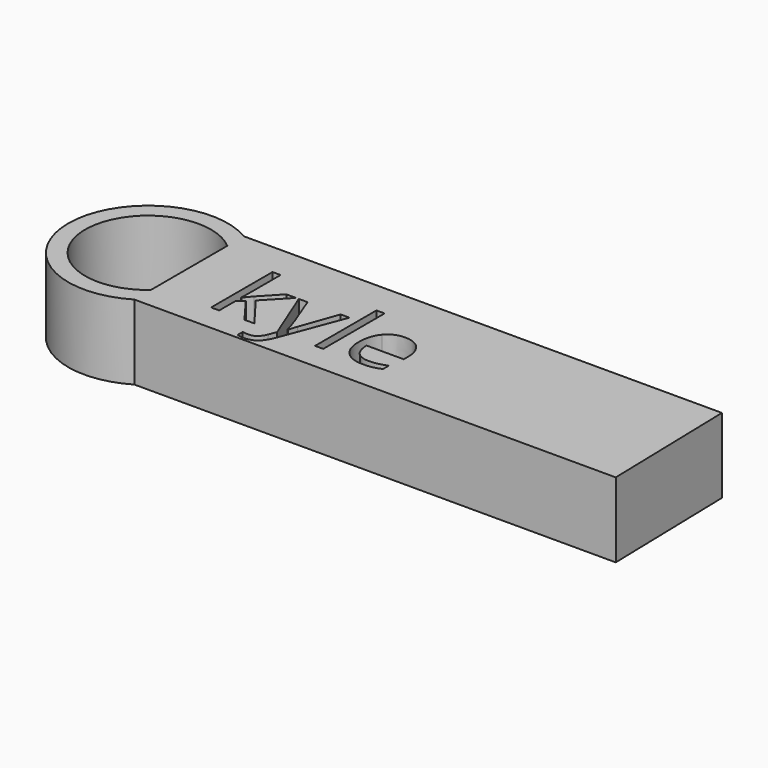
from build123d import *

# Parameters (mm, degrees)
F0_W     = 1.390167144
F0_H     = 13.0257857824
F1_DEPTH = 12.7


with BuildPart() as f1:
    # F0 (on Top) → F1 (new body)
    with BuildSketch(Plane.XY):
        with BuildLine():
            Line((-43.1278555505, 8.1087965258), (-43.1278555505, 11.6189617885))
            ThreePointArc((-43.1278555505, 11.6189617885), (-63.6173153539, 0), (-43.1278555505, -11.6189617885))
            Line((-43.1278555505, -11.6189617885), (-43.1278555505, -8.1087965258))
            ThreePointArc((-43.1278555505, -8.1087965258), (-60.7580848758, 0), (-43.1278555505, 8.1087965258))
        make_face()
        Polygon((37.9903619809, 11.6189617885), (-43.1278555505, 11.6189617885), (-43.1278555505, 8.1087965258), (-43.1278555505, -8.1087965258), (-43.1278555505, -11.6189617885), (38.5659746826, -11.6189617885), align=None)
        with BuildLine():
            Line((-22.5185390528, -7.0921576955), (-26.2202943379, 2.1327664737))
            Line((-26.2202943379, 2.1327664737), (-24.7283423163, 2.1327664737))
            Line((-24.7283423163, 2.1327664737), (-22.7194302586, -3.0984405247))
            add(Edge.make_bspline(
                [(-22.7194302586, -3.0984405247), (-22.0605071037, -4.8903900802), (-21.899794139, -5.6859192551)],
                knots=[0, 0, 0, 1, 1, 1], degree=2))
            Line((-21.899794139, -5.6859192551), (-21.8328304038, -5.6859192551))
            add(Edge.make_bspline(
                [(-21.8328304038, -5.6859192551), (-21.7256884274, -5.2573513494), (-21.377477004, -4.223431277)],
                knots=[0, 0, 0, 1, 1, 1], degree=2))
            add(Edge.make_bspline(
                [(-21.377477004, -4.223431277), (-21.0292655807, -3.1895112047), (-19.1033885547, 2.1327664737)],
                knots=[0, 0, 0, 1, 1, 1], degree=2))
            Line((-19.1033885547, 2.1327664737), (-17.6141150825, 2.1327664737))
            Line((-17.6141150825, 2.1327664737), (-21.5569398145, -8.3135762266))
            add(Edge.make_bspline(
                [(-21.5569398145, -8.3135762266), (-22.1435421354, -9.8617777858), (-22.9256785632, -10.5113260178)],
                knots=[0, 0, 0, 1, 1, 1], degree=2))
            add(Edge.make_bspline(
                [(-22.9256785632, -10.5113260178), (-23.707814991, -11.1608742498), (-24.8461984904, -11.1608742498)],
                knots=[0, 0, 0, 1, 1, 1], degree=2))
            add(Edge.make_bspline(
                [(-24.8461984904, -11.1608742498), (-25.4836932501, -11.1608742498), (-26.1024381638, -11.0162325816)],
                knots=[0, 0, 0, 1, 1, 1], degree=2))
            Line((-26.1024381638, -11.0162325816), (-26.1024381638, -9.9046345763))
            add(Edge.make_bspline(
                [(-26.1024381638, -9.9046345763), (-25.6417276653, -10.0037409045), (-25.0738751903, -10.0037409045)],
                knots=[0, 0, 0, 1, 1, 1], degree=2))
            add(Edge.make_bspline(
                [(-25.0738751903, -10.0037409045), (-23.6408512558, -10.0037409045), (-23.0301419902, -8.3966112583)],
                knots=[0, 0, 0, 1, 1, 1], degree=2))
            Line((-23.0301419902, -8.3966112583), (-22.5185390528, -7.0921576955))
        make_face(mode=Mode.SUBTRACT)
        with BuildLine():
            Line((-32.4532788157, -2.3457681404), (-32.3863150805, -2.3457681404))
            add(Edge.make_bspline(
                [(-32.3863150805, -2.3457681404), (-32.0273894595, -1.834165203), (-31.2907883716, -1.0064934352)],
                knots=[0, 0, 0, 1, 1, 1], degree=2))
            Line((-31.2907883716, -1.0064934352), (-28.3283127238, 2.1327664737))
            Line((-28.3283127238, 2.1327664737), (-26.6783262871, 2.1327664737))
            Line((-26.6783262871, 2.1327664737), (-30.3961528686, -1.775237116))
            Line((-30.3961528686, -1.775237116), (-26.4185069943, -7.0412652567))
            Line((-26.4185069943, -7.0412652567), (-28.1006360239, -7.0412652567))
            Line((-28.1006360239, -7.0412652567), (-31.3416808104, -2.7046937614))
            Line((-31.3416808104, -2.7046937614), (-32.3863150805, -3.6100434621))
            Line((-32.3863150805, -3.6100434621), (-32.3863150805, -7.0412652567))
            Line((-32.3863150805, -7.0412652567), (-33.760410928, -7.0412652567))
            Line((-33.760410928, -7.0412652567), (-33.760410928, 5.9845205257))
            Line((-33.760410928, 5.9845205257), (-32.3863150805, 5.9845205257))
            Line((-32.3863150805, 5.9845205257), (-32.3863150805, -0.9234584035))
            add(Edge.make_bspline(
                [(-32.3863150805, -0.9234584035), (-32.3863150805, -1.3814903527), (-32.4532788157, -2.3457681404)],
                knots=[0, 0, 0, 1, 1, 1], degree=2))
        make_face(mode=Mode.SUBTRACT)
        with Locations((-15.4297580384, -0.5283723655)):
            Rectangle(F0_W, F0_H, mode=Mode.SUBTRACT)
        with BuildLine():
            add(Edge.make_bspline(
                [(-6.3267078674, -7.0707293002), (-6.982952473, -7.2100138696), (-7.9124091183, -7.2100138696)],
                knots=[0, 0, 0, 1, 1, 1], degree=2))
            add(Edge.make_bspline(
                [(-7.9124091183, -7.2100138696), (-9.9454281208, -7.2100138696), (-11.1226505866, -5.9698454926)],
                knots=[0, 0, 0, 1, 1, 1], degree=2))
            add(Edge.make_bspline(
                [(-11.1226505866, -5.9698454926), (-12.2998730524, -4.7296771156), (-12.2998730524, -2.5305880497)],
                knots=[0, 0, 0, 1, 1, 1], degree=2))
            add(Edge.make_bspline(
                [(-12.2998730524, -2.5305880497), (-12.2998730524, -0.3100705886), (-11.207024893, 0.995722249)],
                knots=[0, 0, 0, 1, 1, 1], degree=2))
            add(Edge.make_bspline(
                [(-11.207024893, 0.995722249), (-10.1141767336, 2.3015150865), (-8.2713347393, 2.3015150865)],
                knots=[0, 0, 0, 1, 1, 1], degree=2))
            add(Edge.make_bspline(
                [(-8.2713347393, 2.3015150865), (-6.5490274685, 2.3015150865), (-5.5445714396, 1.1671494112)],
                knots=[0, 0, 0, 1, 1, 1], degree=2))
            add(Edge.make_bspline(
                [(-5.5445714396, 1.1671494112), (-4.5401154107, 0.032783736), (-4.5401154107, -1.8261295548)],
                knots=[0, 0, 0, 1, 1, 1], degree=2))
            Line((-4.5401154107, -1.8261295548), (-4.5401154107, -2.7046937614))
            Line((-4.5401154107, -2.7046937614), (-10.8588134697, -2.7046937614))
            add(Edge.make_bspline(
                [(-10.8588134697, -2.7046937614), (-10.8159566791, -4.3198590558), (-10.0418558995, -5.1569057465)],
                knots=[0, 0, 0, 1, 1, 1], degree=2))
            add(Edge.make_bspline(
                [(-10.0418558995, -5.1569057465), (-9.26775512, -5.9939524373), (-7.8615166795, -5.9939524373)],
                knots=[0, 0, 0, 1, 1, 1], degree=2))
            add(Edge.make_bspline(
                [(-7.8615166795, -5.9939524373), (-6.3802788556, -5.9939524373), (-4.9338621741, -5.3752075235)],
                knots=[0, 0, 0, 1, 1, 1], degree=2))
            Line((-4.9338621741, -5.3752075235), (-4.9338621741, -6.6153759005))
            add(Edge.make_bspline(
                [(-4.9338621741, -6.6153759005), (-5.6704632619, -6.9314447309), (-6.3267078674, -7.0707293002)],
                knots=[0, 0, 0, 1, 1, 1], degree=2))
        make_face(mode=Mode.SUBTRACT)
    extrude(amount=F1_DEPTH)


solid = f1.part
